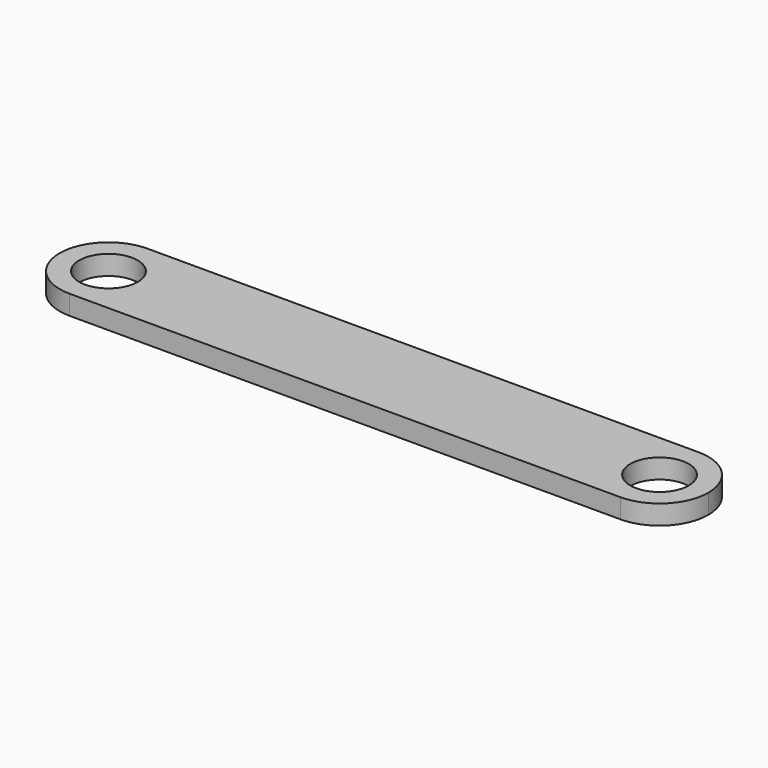
from build123d import *

# Parameters (mm, degrees)
F0_W     = 133
F0_H     = 20
F1_DEPTH = 4
F2_R     = 6
F3_DEPTH = 4.001
F4_R     = 9.99999


# Not quite as in the source:
# - a fillet or chamfer is up to 0.001 mm smaller than in the source, because OpenCascade refuses the exact size


with BuildPart() as f1:
    # F0 (on Top) → F1 (new body)
    with BuildSketch(Plane.XY):
        Rectangle(F0_W, F0_H)
    extrude(amount=F1_DEPTH)

    # F2 (on face) → F3 (cut, through all)
    with BuildSketch(Plane.XY.offset(4)):
        with Locations((-56.5, 0)):
            Circle(F2_R)
        with Locations((56.5, 0)):
            Circle(F2_R)
    extrude(amount=-F3_DEPTH, mode=Mode.SUBTRACT)

    # F4 (radius 10 in the source; OpenCascade refuses exactly that, so slightly less here)
    f4_edges = [f1.edges().sort_by_distance(p)[0] for p in [
        (-66.5, -10, 2),
        (-66.5, 10, 2),
        (66.5, -10, 2),
        (66.5, 10, 2),
    ]]
    fillet(f4_edges, radius=F4_R)


solid = f1.part
